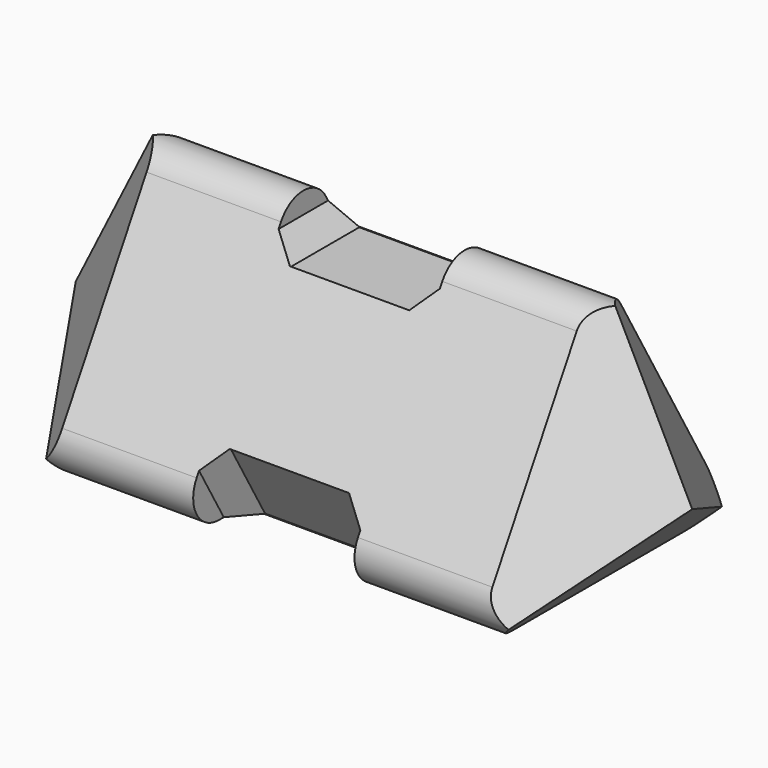
from build123d import *

# Parameters (mm, degrees)
F1_DEPTH    = 20
F4_T1_DEPTH = 32.9903810568
F6_START    = 9.5
F5_W        = 7.5
F5_H        = 4
F6_DEPTH    = 10.5
F8_START    = -9.5
F7_W        = 7.5
F7_H        = 4
F8_DEPTH    = 15.5
F10_START   = -9.5
F9_W        = 7.5
F9_H        = 4
F10_DEPTH   = 10.5
F11_SIZE    = 1


# Not quite as in the source:
# - a fillet or chamfer that OpenCascade refuses, or shapes differently, is made with other operations: its cross-section is extruded or revolved along the edge and cut away or added
# - an extrude whose draft closes it to a point is written as a loft to that point


with BuildPart() as f1:
    # F0 (on Right) → F1 (new body)
    with BuildSketch(Plane.YZ):
        Polygon((-7.5, 0), (7.5, 0), (0, 12.9903810568), align=None)
    extrude(amount=F1_DEPTH)

    # F1_face (on face) → F2 section 0
    with BuildSketch(Plane(origin=(0, 0, 4.3301270189), x_dir=(0, 1, 0), z_dir=(-1, 0, 0)), mode=Mode.PRIVATE) as f2_s0:
        Polygon((7.5, 4.3301270189), (-7.5, 4.3301270189), (0, -8.6602540378), align=None)
    loft([f2_s0.sketch, Vertex(-4.3301270189, 0, 4.3301270189)], ruled=True)

    # F1_face1 (on face) → F3 section 0
    with BuildSketch(Plane(origin=(20, 0, 4.3301270189), x_dir=(0, 1, 0), z_dir=(1, 0, 0)), mode=Mode.PRIVATE) as f3_s0:
        Polygon((-7.5, -4.3301270189), (7.5, -4.3301270189), (0, 8.6602540378), align=None)
    loft([f3_s0.sketch, Vertex(24.3301270189, 0, 4.3301270189)], ruled=True)

    # F4: fillet of radius 1.5 on 3 edges, made by hand

    # F4_s2 → F4_t1 (cut)
    with BuildSketch(Plane.YZ.offset(-6.4951905284)):
        with BuildLine():
            ThreePointArc((-1.2990381057, 10.7403810568), (0, 11.4903810568), (1.2990381057, 10.7403810568))
            Line((1.2990381057, 10.7403810568), (0, 12.9903810568))
            Line((0, 12.9903810568), (-1.2990381057, 10.7403810568))
        make_face()
        with BuildLine():
            ThreePointArc((-4.9019237886, 0), (-6.2009618943, 0.75), (-6.2009618943, 2.25))
            Line((-6.2009618943, 2.25), (-7.5, 0))
            Line((-7.5, 0), (-4.9019237886, 0))
        make_face()
        with BuildLine():
            ThreePointArc((4.9019237886, 0), (6.2009618943, 0.75), (6.2009618943, 2.25))
            Line((6.2009618943, 2.25), (7.5, 0))
            Line((7.5, 0), (4.9019237886, 0))
        make_face()
    extrude(amount=F4_T1_DEPTH, mode=Mode.SUBTRACT)

    # F5 (on Top) → F6 (cut)
    with BuildSketch(Plane.XY.offset(F6_START)):
        with Locations((10, -0.0009618943)):
            Rectangle(F5_W, F5_H)
    extrude(amount=F6_DEPTH, mode=Mode.SUBTRACT)

    # F7 (on face) → F8 (cut)
    with BuildSketch(Plane(origin=(0, -5.625, 3.2475952642), x_dir=(1, 0, 0), z_dir=(0, -0.8660254038, 0.5)).offset(F8_START)):
        with Locations((10, 3.7480762114)):
            Rectangle(F7_W, F7_H)
    extrude(amount=-F8_DEPTH, mode=Mode.SUBTRACT)

    # F9 (on face) → F10 (cut)
    with BuildSketch(Plane(origin=(0, 5.625, 3.2475952642), x_dir=(-1, 0, 0), z_dir=(0, 0.8660254038, 0.5)).offset(F10_START)):
        with Locations((-10, 3.7519237886)):
            Rectangle(F9_W, F9_H)
    extrude(amount=-F10_DEPTH, mode=Mode.SUBTRACT)

    # F11
    f11_edges = [f1.edges().sort_by_distance(p)[0] for p in [
        (6.25, 4.476279, 1.743524),
        (13.75, 4.476279, 1.743524),
        (6.25, -4.478203, 1.746857),
        (13.75, -4.478203, 1.746857),
        (6.25, -0.000962, 9.5),
        (13.75, -0.000962, 9.5),
    ]]
    chamfer(f11_edges, length=F11_SIZE)


solid = f1.part
